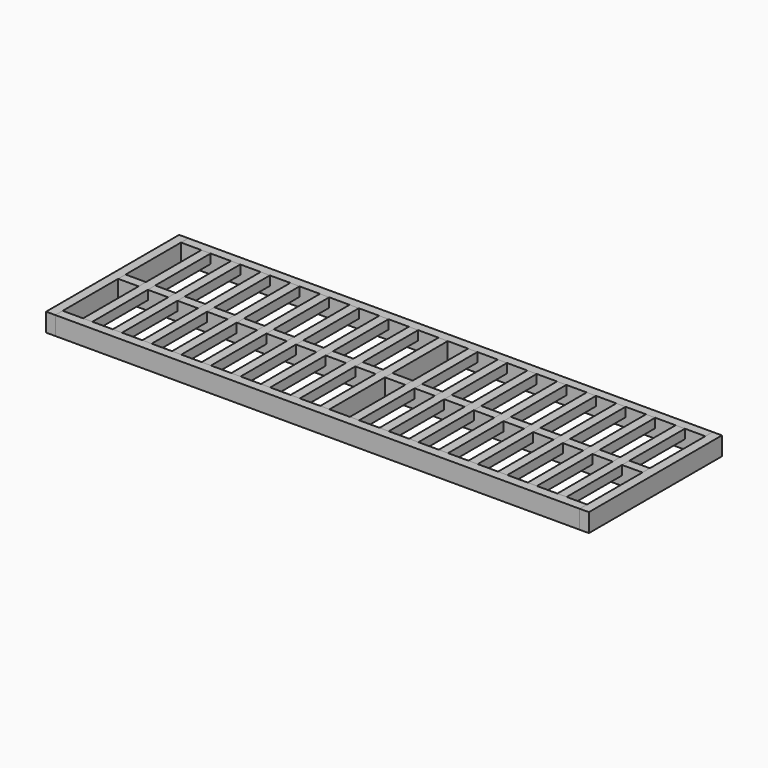
from build123d import *

# Parameters (mm, degrees)
F0_W     = 50.8
F0_H     = 381
F0_H_2   = 50.8
F1_DEPTH = 50.8
F0_W_2   = 112.17275
F2_DEPTH = 101.6
F3_DEPTH = 101.6
F0_W_3   = 112.268
F4_DEPTH = 101.6
F5_DEPTH = 50.8


# Not quite as in the source:
# - a feature names something its author has since deleted; it is built from what else it names


with BuildPart() as f1:
    # F0 (on Top) → F1 (new body)
    with BuildSketch(Plane.XY):
        with Locations((1303.782, 215.9)):
            Rectangle(F0_W, F0_H)
        with Locations((1303.782, -215.9)):
            Rectangle(F0_W, F0_H)
        with Locations((1303.782, 0)):
            Rectangle(F0_W, F0_H_2)
    extrude(amount=-F1_DEPTH)


with BuildPart() as f1b:
    # F0 (on Top) → F1, piece 2 (new body)
    with BuildSketch(Plane.XY):
        with Locations((1140.80925, -215.9)):
            Rectangle(F0_W, F0_H)
        with Locations((1140.80925, 0)):
            Rectangle(F0_W, F0_H_2)
        with Locations((1140.80925, 215.9)):
            Rectangle(F0_W, F0_H)
    extrude(amount=-F1_DEPTH)


with BuildPart() as f1c:
    # F0 (on Top) → F1, piece 3 (new body)
    with BuildSketch(Plane.XY):
        with Locations((977.8365, -215.9)):
            Rectangle(F0_W, F0_H)
        with Locations((977.8365, 0)):
            Rectangle(F0_W, F0_H_2)
        with Locations((977.8365, 215.9)):
            Rectangle(F0_W, F0_H)
    extrude(amount=-F1_DEPTH)


with BuildPart() as f1d:
    # F0 (on Top) → F1, piece 4 (new body)
    with BuildSketch(Plane.XY):
        with Locations((651.891, 0)):
            Rectangle(F0_W, F0_H_2)
        with Locations((651.891, 215.9)):
            Rectangle(F0_W, F0_H)
        with Locations((651.891, -215.9)):
            Rectangle(F0_W, F0_H)
    extrude(amount=-F1_DEPTH)


with BuildPart() as f1e:
    # F0 (on Top) → F1, piece 5 (new body)
    with BuildSketch(Plane.XY):
        with Locations((488.91825, 0)):
            Rectangle(F0_W, F0_H_2)
        with Locations((488.91825, 215.9)):
            Rectangle(F0_W, F0_H)
        with Locations((488.91825, -215.9)):
            Rectangle(F0_W, F0_H)
    extrude(amount=-F1_DEPTH)


with BuildPart() as f1f:
    # F0 (on Top) → F1, piece 6 (new body)
    with BuildSketch(Plane.XY):
        with Locations((325.9455, 0)):
            Rectangle(F0_W, F0_H_2)
        with Locations((325.9455, -215.9)):
            Rectangle(F0_W, F0_H)
        with Locations((325.9455, 215.9)):
            Rectangle(F0_W, F0_H)
    extrude(amount=-F1_DEPTH)


with BuildPart() as f1g:
    # F0 (on Top) → F1, piece 7 (new body)
    with BuildSketch(Plane.XY):
        with Locations((162.97275, -215.9)):
            Rectangle(F0_W, F0_H)
        with Locations((162.97275, 215.9)):
            Rectangle(F0_W, F0_H)
        with Locations((162.97275, 0)):
            Rectangle(F0_W, F0_H_2)
    extrude(amount=-F1_DEPTH)


with BuildPart() as f1h:
    # F0 (on Top) → F1, piece 8 (new body)
    with BuildSketch(Plane.XY):
        with Locations((0, 215.9)):
            Rectangle(F0_W, F0_H)
        with Locations((0, -215.9)):
            Rectangle(F0_W, F0_H)
        Rectangle(F0_W, F0_H_2)
    extrude(amount=-F1_DEPTH)

    # F0 (on Top) → F2, piece 2 (join)
    with BuildSketch(Plane.XY):
        with Locations((0, 215.9)):
            Rectangle(F0_W, F0_H)
        with Locations((0, -215.9)):
            Rectangle(F0_W, F0_H)
    extrude(amount=-F2_DEPTH)


with BuildPart() as f1i:
    # F0 (on Top) → F1, piece 9 (new body)
    with BuildSketch(Plane.XY):
        with Locations((-162.97275, -215.9)):
            Rectangle(F0_W, F0_H)
        with Locations((-162.97275, 0)):
            Rectangle(F0_W, F0_H_2)
        with Locations((-162.97275, 215.9)):
            Rectangle(F0_W, F0_H)
    extrude(amount=-F1_DEPTH)


with BuildPart() as f1j:
    # F0 (on Top) → F1, piece 10 (new body)
    with BuildSketch(Plane.XY):
        with Locations((-488.91825, -215.9)):
            Rectangle(F0_W, F0_H)
        with Locations((-488.91825, 215.9)):
            Rectangle(F0_W, F0_H)
        with Locations((-488.91825, 0)):
            Rectangle(F0_W, F0_H_2)
    extrude(amount=-F1_DEPTH)


with BuildPart() as f1k:
    # F0 (on Top) → F1, piece 11 (new body)
    with BuildSketch(Plane.XY):
        with Locations((-814.86375, 0)):
            Rectangle(F0_W, F0_H_2)
        with Locations((-814.86375, -215.9)):
            Rectangle(F0_W, F0_H)
        with Locations((-814.86375, 215.9)):
            Rectangle(F0_W, F0_H)
    extrude(amount=-F1_DEPTH)


with BuildPart() as f1l:
    # F0 (on Top) → F1, piece 12 (new body)
    with BuildSketch(Plane.XY):
        with Locations((-977.8365, -215.9)):
            Rectangle(F0_W, F0_H)
        with Locations((-977.8365, 215.9)):
            Rectangle(F0_W, F0_H)
        with Locations((-977.8365, 0)):
            Rectangle(F0_W, F0_H_2)
    extrude(amount=-F1_DEPTH)


with BuildPart() as f1m:
    # F0 (on Top) → F1, piece 13 (new body)
    with BuildSketch(Plane.XY):
        with Locations((-1140.80925, -215.9)):
            Rectangle(F0_W, F0_H)
        with Locations((-1140.80925, 215.9)):
            Rectangle(F0_W, F0_H)
        with Locations((-1140.80925, 0)):
            Rectangle(F0_W, F0_H_2)
    extrude(amount=-F1_DEPTH)


with BuildPart() as f1n:
    # F0 (on Top) → F1, piece 14 (new body)
    with BuildSketch(Plane.XY):
        with Locations((-1303.782, -215.9)):
            Rectangle(F0_W, F0_H)
        with Locations((-1303.782, 0)):
            Rectangle(F0_W, F0_H_2)
        with Locations((-1303.782, 215.9)):
            Rectangle(F0_W, F0_H)
    extrude(amount=-F1_DEPTH)


with BuildPart() as f1o:
    # F0 (on Top) → F1, piece 15 (new body)
    with BuildSketch(Plane.XY):
        with Locations((-325.9455, -215.9)):
            Rectangle(F0_W, F0_H)
        with Locations((-325.9455, 0)):
            Rectangle(F0_W, F0_H_2)
        with Locations((-325.9455, 215.9)):
            Rectangle(F0_W, F0_H)
    extrude(amount=-F1_DEPTH)


with BuildPart() as f1p:
    # F0 (on Top) → F1, piece 16 (new body)
    with BuildSketch(Plane.XY):
        with Locations((-651.891, -215.9)):
            Rectangle(F0_W, F0_H)
        with Locations((-651.891, 215.9)):
            Rectangle(F0_W, F0_H)
        with Locations((-651.891, 0)):
            Rectangle(F0_W, F0_H_2)
    extrude(amount=-F1_DEPTH)


with BuildPart() as f1q:
    # F0 (on Top) → F1, piece 17 (new body)
    with BuildSketch(Plane.XY):
        with Locations((814.86375, -215.9)):
            Rectangle(F0_W, F0_H)
        with Locations((814.86375, 215.9)):
            Rectangle(F0_W, F0_H)
        with Locations((814.86375, 0)):
            Rectangle(F0_W, F0_H_2)
    extrude(amount=-F1_DEPTH)


with BuildPart() as f2:
    # F0 (on Top) → F2 (new body)
    with BuildSketch(Plane.XY):
        with Locations((1303.782, 0)):
            Rectangle(F0_W, F0_H_2)
        with Locations((1222.295625, 0)):
            Rectangle(F0_W_2, F0_H_2)
    extrude(amount=-F2_DEPTH)

    # F0 (on Top) → F4 (join)
    with BuildSketch(Plane.XY):
        with Locations((1385.316, 0)):
            Rectangle(F0_W_3, F0_H_2)
        with Locations((1140.80925, 0)):
            Rectangle(F0_W, F0_H_2)
        with Locations((977.8365, 0)):
            Rectangle(F0_W, F0_H_2)
        with Locations((1059.322875, 0)):
            Rectangle(F0_W_2, F0_H_2)
        with Locations((896.350125, 0)):
            Rectangle(F0_W_2, F0_H_2)
        with Locations((814.86375, 0)):
            Rectangle(F0_W, F0_H_2)
        with Locations((570.404625, 0)):
            Rectangle(F0_W_2, F0_H_2)
        with Locations((-325.9455, 0)):
            Rectangle(F0_W, F0_H_2)
        with Locations((325.9455, 0)):
            Rectangle(F0_W, F0_H_2)
        with Locations((407.431875, 0)):
            Rectangle(F0_W_2, F0_H_2)
        with Locations((651.891, 0)):
            Rectangle(F0_W, F0_H_2)
        with Locations((-244.459125, 0)):
            Rectangle(F0_W_2, F0_H_2)
        with Locations((-896.350125, 0)):
            Rectangle(F0_W_2, F0_H_2)
        with Locations((-977.8365, 0)):
            Rectangle(F0_W, F0_H_2)
        with Locations((-1222.295625, 0)):
            Rectangle(F0_W_2, F0_H_2)
        with Locations((-162.97275, 0)):
            Rectangle(F0_W, F0_H_2)
        with Locations((81.486375, 0)):
            Rectangle(F0_W_2, F0_H_2)
        with Locations((-81.486375, 0)):
            Rectangle(F0_W_2, F0_H_2)
        with Locations((-1059.322875, 0)):
            Rectangle(F0_W_2, F0_H_2)
        with Locations((244.459125, 0)):
            Rectangle(F0_W_2, F0_H_2)
        with Locations((-1385.316, 0)):
            Rectangle(F0_W_3, F0_H_2)
        with Locations((-1140.80925, 0)):
            Rectangle(F0_W, F0_H_2)
        with Locations((162.97275, 0)):
            Rectangle(F0_W, F0_H_2)
        with Locations((-814.86375, 0)):
            Rectangle(F0_W, F0_H_2)
        Rectangle(F0_W, F0_H_2)
        with Locations((-488.91825, 0)):
            Rectangle(F0_W, F0_H_2)
        with Locations((-407.431875, 0)):
            Rectangle(F0_W_2, F0_H_2)
        with Locations((733.377375, 0)):
            Rectangle(F0_W_2, F0_H_2)
        with Locations((-1303.782, 0)):
            Rectangle(F0_W, F0_H_2)
        with Locations((-570.404625, 0)):
            Rectangle(F0_W_2, F0_H_2)
        with Locations((-733.377375, 0)):
            Rectangle(F0_W_2, F0_H_2)
        with Locations((-651.891, 0)):
            Rectangle(F0_W, F0_H_2)
        with Locations((488.91825, 0)):
            Rectangle(F0_W, F0_H_2)
    extrude(amount=-F4_DEPTH)

    # F0 (on Top) → F5 (cut)
    with BuildSketch(Plane.XY):
        with Locations((1303.782, 0)):
            Rectangle(F0_W, F0_H_2)
        with Locations((1140.80925, 0)):
            Rectangle(F0_W, F0_H_2)
        with Locations((977.8365, 0)):
            Rectangle(F0_W, F0_H_2)
        with Locations((814.86375, 0)):
            Rectangle(F0_W, F0_H_2)
        with Locations((651.891, 0)):
            Rectangle(F0_W, F0_H_2)
        with Locations((488.91825, 0)):
            Rectangle(F0_W, F0_H_2)
        with Locations((325.9455, 0)):
            Rectangle(F0_W, F0_H_2)
        with Locations((162.97275, 0)):
            Rectangle(F0_W, F0_H_2)
        Rectangle(F0_W, F0_H_2)
        with Locations((-162.97275, 0)):
            Rectangle(F0_W, F0_H_2)
        with Locations((-325.9455, 0)):
            Rectangle(F0_W, F0_H_2)
        with Locations((-488.91825, 0)):
            Rectangle(F0_W, F0_H_2)
        with Locations((-651.891, 0)):
            Rectangle(F0_W, F0_H_2)
        with Locations((-814.86375, 0)):
            Rectangle(F0_W, F0_H_2)
        with Locations((-977.8365, 0)):
            Rectangle(F0_W, F0_H_2)
        with Locations((-1140.80925, 0)):
            Rectangle(F0_W, F0_H_2)
        with Locations((-1303.782, 0)):
            Rectangle(F0_W, F0_H_2)
    extrude(amount=-F5_DEPTH, mode=Mode.SUBTRACT)


with BuildPart() as f3:
    # F0 (on Top) → F3 (new body)
    with BuildSketch(Plane.XY):
        Polygon((-1441.45, 406.4), (-1441.45, 457.2), (-1492.25, 457.2), (-1492.25, -457.2), (-1441.45, -457.2), (-1441.45, -406.4), (-1441.45, -25.4), (-1441.45, 25.4), align=None)
    extrude(amount=-F3_DEPTH)


with BuildPart() as f3b:
    # F0 (on Top) → F3, piece 2 (new body)
    with BuildSketch(Plane.XY):
        Polygon((1492.25, -457.2), (1492.25, 457.2), (1441.45, 457.2), (1441.45, 406.4), (1441.45, 25.4), (1441.45, -25.4), (1441.45, -406.4), (1441.45, -457.2), align=None)
    extrude(amount=-F3_DEPTH)


with BuildPart() as f4:
    # F0 (on Top) → F4, piece 2 (new body)
    with BuildSketch(Plane.XY):
        Polygon((1441.45, 406.4), (1441.45, 457.2), (-1441.45, 457.2), (-1441.45, 406.4), (-1329.182, 406.4), (-1278.382, 406.4), (-1166.20925, 406.4), (-1115.40925, 406.4), (-1003.2365, 406.4), (-952.4365, 406.4), (-840.26375, 406.4), (-789.46375, 406.4), (-677.291, 406.4), (-626.491, 406.4), (-514.31825, 406.4), (-463.51825, 406.4), (-351.3455, 406.4), (-300.5455, 406.4), (-188.37275, 406.4), (-137.57275, 406.4), (-25.4, 406.4), (25.4, 406.4), (137.57275, 406.4), (188.37275, 406.4), (300.5455, 406.4), (351.3455, 406.4), (463.51825, 406.4), (514.31825, 406.4), (626.491, 406.4), (677.291, 406.4), (789.46375, 406.4), (840.26375, 406.4), (952.4365, 406.4), (1003.2365, 406.4), (1115.40925, 406.4), (1166.20925, 406.4), (1278.382, 406.4), (1329.182, 406.4), align=None)
    extrude(amount=-F4_DEPTH)


with BuildPart() as f4b:
    # F0 (on Top) → F4, piece 3 (new body)
    with BuildSketch(Plane.XY):
        Polygon((-1441.45, -457.2), (1441.45, -457.2), (1441.45, -406.4), (1329.182, -406.4), (1278.382, -406.4), (1166.20925, -406.4), (1115.40925, -406.4), (1003.2365, -406.4), (952.4365, -406.4), (840.26375, -406.4), (789.46375, -406.4), (677.291, -406.4), (626.491, -406.4), (514.31825, -406.4), (463.51825, -406.4), (351.3455, -406.4), (300.5455, -406.4), (188.37275, -406.4), (137.57275, -406.4), (25.4, -406.4), (-25.4, -406.4), (-137.57275, -406.4), (-188.37275, -406.4), (-300.5455, -406.4), (-351.3455, -406.4), (-463.51825, -406.4), (-514.31825, -406.4), (-626.491, -406.4), (-677.291, -406.4), (-789.46375, -406.4), (-840.26375, -406.4), (-952.4365, -406.4), (-1003.2365, -406.4), (-1115.40925, -406.4), (-1166.20925, -406.4), (-1278.382, -406.4), (-1329.182, -406.4), (-1441.45, -406.4), align=None)
    extrude(amount=-F4_DEPTH)


solid = Compound([f1.part, f1b.part, f1c.part, f1d.part, f1e.part, f1f.part, f1g.part, f1h.part, f1i.part, f1j.part, f1k.part, f1l.part, f1m.part, f1n.part, f1o.part, f1p.part, f1q.part, f2.part, f3.part, f3b.part, f4.part, f4b.part])
